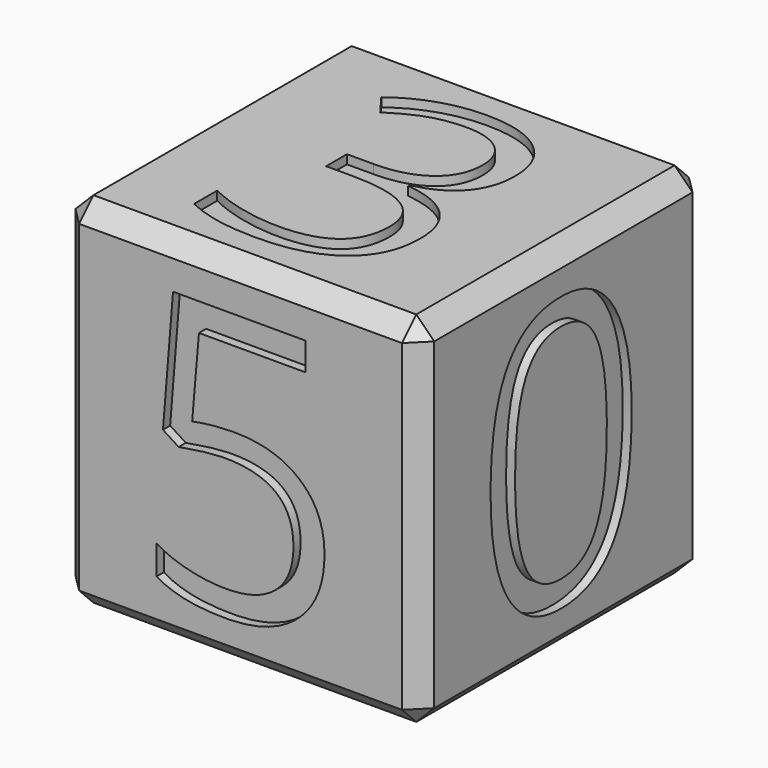
from build123d import *

# Parameters (mm, degrees)
F0_W          = 50.8
F0_H          = 50.8
F1_DEPTH      = 25.4
F1_DEPTH_BACK = 25.4
F2_SIZE       = 2.54
F3_TEXT_SIZE  = 52.9166666667
F4_DEPTH      = 1.27
F5_TEXT_SIZE  = 52.9166666667
F6_DEPTH      = 1.27
F7_TEXT_SIZE  = 52.9166666667
F8_DEPTH      = 1.27
F9_TEXT_SIZE  = 52.9166666667
F10_DEPTH     = 1.27
F11_TEXT_SIZE = 52.9166666667
F12_DEPTH     = 1.27
F13_TEXT_SIZE = 52.9166666667
F14_DEPTH     = 1.27


# Not quite as in the source:
# - Text() gives the source's letters only with a copy of the font that has no kerning and outlines rounded to 1/6400 em; it was checked with that copy


with BuildPart() as f1:
    # F0 (on Top) → F1 (new body, two sides)
    with BuildSketch(Plane.XY) as f1_sk:
        Rectangle(F0_W, F0_H)
    extrude(amount=F1_DEPTH)
    extrude(f1_sk.sketch, amount=-F1_DEPTH_BACK)

    # F2
    f2_edges = [f1.edges().sort_by_distance(p)[0] for p in [
        (-25.4, 0, 25.4),
        (-25.4, -25.4, 0),
        (-25.4, 0, -25.4),
        (-25.4, 25.4, 0),
        (25.4, 0, 25.4),
        (0, 25.4, 25.4),
        (0, -25.4, 25.4),
        (0, 25.4, -25.4),
        (25.4, 25.4, 0),
        (25.4, -25.4, 0),
        (25.4, 0, -25.4),
        (0, -25.4, -25.4),
    ]]
    chamfer(f2_edges, length=F2_SIZE)

    # F3 (on face) → F4 (cut)
    with BuildSketch(Plane.YZ.offset(25.4)):
        with Locations((-15.527734375, -19.05)):
            Text('0', F3_TEXT_SIZE, font='Open Sans', text_align=(TextAlign.LEFT, TextAlign.BOTTOM))
    extrude(amount=-F4_DEPTH, mode=Mode.SUBTRACT)

    # F5 (on face) → F6 (cut)
    with BuildSketch(Plane(origin=(0, 25.4, 0), x_dir=(-1, 0, 0), z_dir=(0, 1, 0))):
        with Locations((-10.9512695313, -19.05)):
            Text('1', F5_TEXT_SIZE, font='Open Sans', text_align=(TextAlign.LEFT, TextAlign.BOTTOM))
    extrude(amount=-F6_DEPTH, mode=Mode.SUBTRACT)

    # F7 (on face) → F8 (cut)
    with BuildSketch(Plane(origin=(0, 0, -25.4), x_dir=(1, 0, 0), z_dir=(0, 0, -1))):
        with Locations((-15.4243815104, -17.7181996551)):
            Text('2', F7_TEXT_SIZE, font='Open Sans', text_align=(TextAlign.LEFT, TextAlign.BOTTOM))
    extrude(amount=-F8_DEPTH, mode=Mode.SUBTRACT)

    # F9 (on face) → F10 (cut)
    with BuildSketch(Plane.XY.offset(25.4)):
        with Locations((-15.2920898438, -19.05)):
            Text('3', F9_TEXT_SIZE, font='Open Sans', text_align=(TextAlign.LEFT, TextAlign.BOTTOM))
    extrude(amount=-F10_DEPTH, mode=Mode.SUBTRACT)

    # F11 (on face) → F12 (cut)
    with BuildSketch(Plane(origin=(-25.4, 0, 0), x_dir=(0, -1, 0), z_dir=(-1, 0, 0))):
        with Locations((-16.3132161458, -19.05)):
            Text('4', F11_TEXT_SIZE, font='Open Sans', text_align=(TextAlign.LEFT, TextAlign.BOTTOM))
    extrude(amount=-F12_DEPTH, mode=Mode.SUBTRACT)

    # F13 (on face) → F14 (cut)
    with BuildSketch(Plane.XZ.offset(25.4)):
        with Locations((-15.3210286458, -19.05)):
            Text('5', F13_TEXT_SIZE, font='Open Sans', text_align=(TextAlign.LEFT, TextAlign.BOTTOM))
    extrude(amount=-F14_DEPTH, mode=Mode.SUBTRACT)


solid = f1.part
